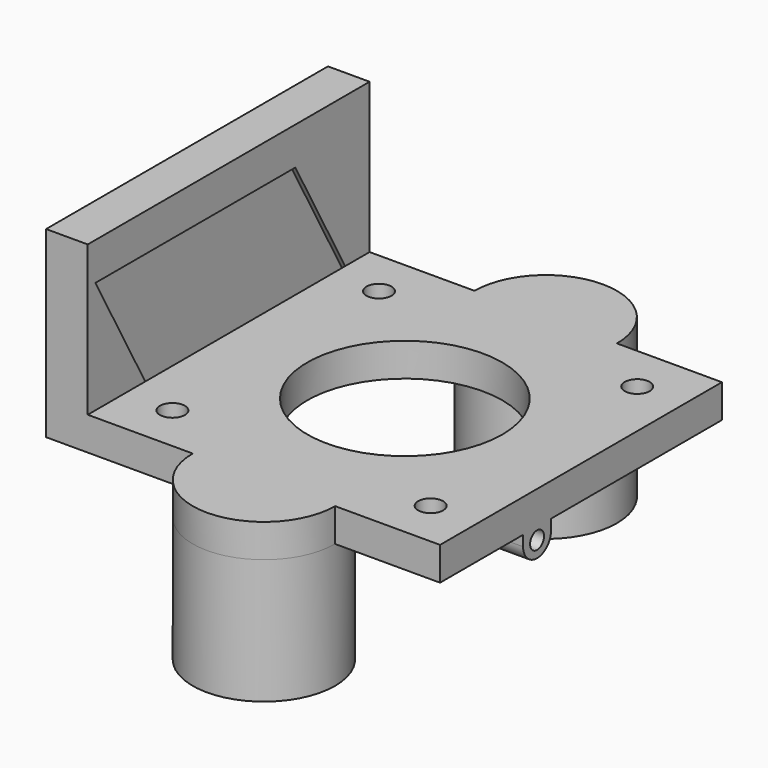
from build123d import *

# Parameters (mm, degrees)
F0_R      = 1.5
F0_R_2    = 11.7126871306
F1_DEPTH  = 4
F2_R      = 4
F3_DEPTH  = 15
F6_DEPTH  = 0.6
F7_W      = 42.3
F7_H      = 22
F8_DEPTH  = 5
F11_R     = 1.0444740365
F12_DEPTH = 5
F14_R     = 1.0444740365
F15_DEPTH = 5
F16_W     = 6.0576063115
F16_H     = 10.3428596631
F16_R     = 1.0444740365
F17_DEPTH = 6
F18_SIZE  = 5.99999
F19_R     = 1.4573614865
F20_DEPTH = 7
F21_W     = 1.9849594682
F21_H     = 5.3345812485
F22_DEPTH = 5
F23_W     = 6.0576063115
F23_H     = 5.2529345267
F24_DEPTH = 1


# Not quite as in the source:
# - a fillet or chamfer is up to 0.001 mm smaller than in the source, because OpenCascade refuses the exact size


with BuildPart() as f1:
    # F0 (on Top) → F1 (new body)
    with BuildSketch(Plane.XY):
        with BuildLine():
            Line((21.15, -21.15), (21.15, 21.15))
            Line((21.15, 21.15), (8.5471369535, 21.15))
            ThreePointArc((8.5471369535, 21.15), (6.0437384995, 27.1937384995), (0, 29.6971369535))
            ThreePointArc((0, 29.6971369535), (-6.0437384995, 27.1937384995), (-8.5471369535, 21.15))
            Line((-8.5471369535, 21.15), (-21.15, 21.15))
            Line((-21.15, 21.15), (-21.15, -21.15))
            Line((-21.15, -21.15), (-8.5471369535, -21.15))
            ThreePointArc((-8.5471369535, -21.15), (0, -29.6971369535), (8.5471369535, -21.15))
            Line((8.5471369535, -21.15), (21.15, -21.15))
        make_face()
        with Locations((-15.5, -15.5)):
            Circle(F0_R, mode=Mode.SUBTRACT)
        with Locations((15.5, -15.5)):
            Circle(F0_R, mode=Mode.SUBTRACT)
        with Locations((-15.5, 15.5)):
            Circle(F0_R, mode=Mode.SUBTRACT)
        Circle(F0_R_2, mode=Mode.SUBTRACT)
        with Locations((15.5, 15.5)):
            Circle(F0_R, mode=Mode.SUBTRACT)
    extrude(amount=F1_DEPTH)

    # F2 (on face) → F3 (join)
    with BuildSketch(Plane(origin=(0, 0, 0), x_dir=(1, 0, 0), z_dir=(0, 0, -1))):
        with BuildLine():
            ThreePointArc((-8.5471369535, 21.15), (0, 12.6028630465), (8.5471369535, 21.15))
            ThreePointArc((8.5471369535, 21.15), (0, 29.6971369535), (-8.5471369535, 21.15))
        make_face()
        with Locations((0, 21.15)):
            Circle(F2_R, mode=Mode.SUBTRACT)
        with BuildLine():
            ThreePointArc((-8.5471369535, -21.15), (0, -29.6971369535), (8.5471369535, -21.15))
            ThreePointArc((8.5471369535, -21.15), (0, -12.6028630465), (-8.5471369535, -21.15))
        make_face()
        with Locations((0, -21.15)):
            Circle(F2_R, mode=Mode.SUBTRACT)
    extrude(amount=F3_DEPTH)

    # F7 (on face) → F8 (join)
    with BuildSketch(Plane(origin=(-21.15, 0, 0), x_dir=(0, -1, 0), z_dir=(-1, 0, 0))):
        with Locations((0, 11)):
            Rectangle(F7_W, F7_H)
    extrude(amount=F8_DEPTH)

    # F9: union 


with BuildPart() as f6:
    # F5 (on offset) → F6 (new body)
    with BuildSketch(Plane(origin=(-21.15, 0, 0), x_dir=(0, -1, 0), z_dir=(-1, 0, 0))):
        Polygon((-10, 17.4662213922), (-20, -0.5337786078), (10, -0.5337786078), (20, 17.4662213922), align=None)
    extrude(amount=F6_DEPTH)


with BuildPart() as f1_1:
    add(f1.part)

    # F10: cut F6
    add(f6.part, mode=Mode.SUBTRACT)

    # F11 (on face) → F12 (join)
    with BuildSketch(Plane.YZ.offset(21.15)):
        with BuildLine():
            Line((-4.4944686815, -1.2040658621), (-4.4944686815, 0))
            Line((-4.4944686815, 0), (-8.6928773671, 0))
            Line((-8.6928773671, 0), (-8.6928773671, -1.2551693944))
            ThreePointArc((-8.6928773671, -1.2551693944), (-6.5681212582, -3.3288219711), (-4.4944686815, -1.2040658621))
        make_face()
        with Locations((-6.5936730243, -1.4166244073)):
            Circle(F11_R, mode=Mode.SUBTRACT)
    extrude(amount=-F12_DEPTH)

    # F14 (on offset) → F15 (join)
    with BuildSketch(Plane(origin=(-17.25, 0, 0), x_dir=(0, -1, 0), z_dir=(-1, 0, 0))):
        with BuildLine():
            Line((8.6928773671, -1.2551693944), (8.6928773671, 0))
            Line((8.6928773671, 0), (4.4944686815, 0))
            Line((4.4944686815, 0), (4.4944686815, -1.2040658621))
            ThreePointArc((4.4944686815, -1.2040658621), (6.5681212582, -3.3288219711), (8.6928773671, -1.2551693944))
        make_face()
        with Locations((6.5936730243, -1.4166244073)):
            Circle(F14_R, mode=Mode.SUBTRACT)
    extrude(amount=-F15_DEPTH)

    # F16 (on face) → F17 (join)
    with BuildSketch(Plane(origin=(-26.15, 0, 0), x_dir=(0, -1, 0), z_dir=(-1, 0, 0))):
        with Locations((6.7643582588, 0.7691108622)):
            Rectangle(F16_W, F16_H)
        with BuildLine():
            ThreePointArc((8.6928773671, -1.2551693944), (6.5681212582, -3.3288219711), (4.4944686815, -1.2040658621))
            Line((4.4944686815, -1.2040658621), (4.4944686815, 0))
            Line((4.4944686815, 0), (8.6928773671, 0))
            Line((8.6928773671, 0), (8.6928773671, -1.2551693944))
        make_face(mode=Mode.SUBTRACT)
        with BuildLine():
            ThreePointArc((8.6928773671, -1.2551693944), (6.5681212582, -3.3288219711), (4.4944686815, -1.2040658621))
            Line((4.4944686815, -1.2040658621), (4.4944686815, 0))
            Line((4.4944686815, 0), (3.735555103, 0))
            Line((3.735555103, 0), (3.735555103, -4.4023189694))
            Line((3.735555103, -4.4023189694), (9.7931614146, -4.4023189694))
            Line((9.7931614146, -4.4023189694), (9.7931614146, 0))
            Line((9.7931614146, 0), (8.6928773671, 0))
            Line((8.6928773671, 0), (8.6928773671, -1.2551693944))
        make_face()
        with BuildLine():
            Line((4.4944686815, 0), (4.4944686815, -1.2040658621))
            ThreePointArc((4.4944686815, -1.2040658621), (6.5681212582, -3.3288219711), (8.6928773671, -1.2551693944))
            Line((8.6928773671, -1.2551693944), (8.6928773671, 0))
            Line((8.6928773671, 0), (4.4944686815, 0))
        make_face()
        with Locations((6.5936730243, -1.4166244073)):
            Circle(F16_R, mode=Mode.SUBTRACT)
    extrude(amount=F17_DEPTH)

    # F18 (size 6 in the source; OpenCascade refuses exactly that, so slightly less here)
    f18_edges = [f1_1.edges().sort_by_distance(p)[0] for p in [
        (-32.15, -6.764358, 5.940541),
    ]]
    chamfer(f18_edges, length=F18_SIZE)

    # F19 (on face) → F20 (cut)
    with BuildSketch(Plane(origin=(-32.15, 0, 0), x_dir=(0, -1, 0), z_dir=(-1, 0, 0))):
        with Locations((6.5936730243, -1.4166244073)):
            Circle(F19_R)
    extrude(amount=-F20_DEPTH, mode=Mode.SUBTRACT)

    # F21 (on face) → F22 (cut)
    with BuildSketch(Plane(origin=(0, 0, -4.4023189694), x_dir=(1, 0, 0), z_dir=(0, 0, -1))):
        with Locations((-29.0259411559, 6.7643583752)):
            Rectangle(F21_W, F21_H)
    extrude(amount=-F22_DEPTH, mode=Mode.SUBTRACT)

    # F23 (on face) → F24 (cut)
    with BuildSketch(Plane.YZ.offset(-26.15)):
        with Locations((-6.7643582588, -2.6264672633)):
            Rectangle(F23_W, F23_H)
    extrude(amount=-F24_DEPTH, mode=Mode.SUBTRACT)


solid = f1_1.part
